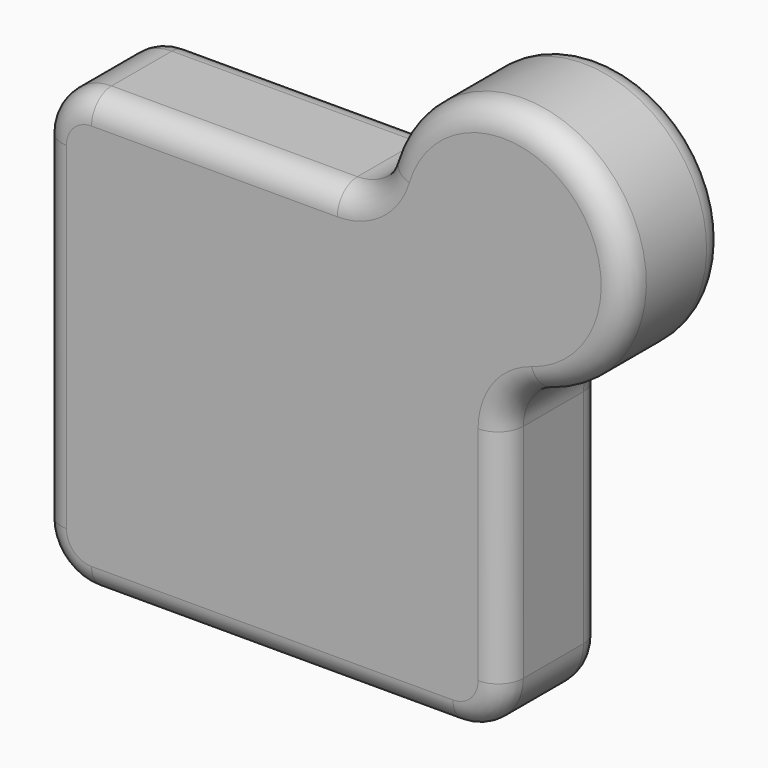
from build123d import *

# Parameters (mm, degrees)
F1_DEPTH = 25
F2_R     = 5


# Not quite as in the source:
# - the program builds the solid bodies; features that only make, move or delete a surface that nothing else refers to are left out


with BuildPart() as f1:
    # F0 (on Front) → F1 (new body)
    with BuildSketch(Plane.XZ):
        with BuildLine():
            ThreePointArc((22.5237740783, 50.7157030305), (18.9120996382, 45.5821277938), (12.9524584639, 43.6122384452))
            Line((12.9524584639, 43.6122384452), (-35.9964722395, 43.6122384452))
            ThreePointArc((-35.9964722395, 43.6122384452), (-43.0675400514, 40.6833062571), (-45.9964722395, 33.6122384452))
            Line((-45.9964722395, 33.6122384452), (-45.9964722395, -33.6122384452))
            ThreePointArc((-45.9964722395, -33.6122384452), (-43.0675400514, -40.6833062571), (-35.9964722395, -43.6122384452))
            Line((-35.9964722395, -43.6122384452), (35.9964722395, -43.6122384452))
            ThreePointArc((35.9964722395, -43.6122384452), (43.0675400514, -40.6833062571), (45.9964722395, -33.6122384452))
            Line((45.9964722395, -33.6122384452), (45.9964722395, 10.5682246696))
            ThreePointArc((45.9964722395, 10.5682246696), (47.9663615881, 16.5278658439), (53.0999368248, 20.139540284))
            ThreePointArc((53.0999368248, 20.139540284), (63.3375617105, 60.9533279162), (22.5237740783, 50.7157030305))
        make_face()
    extrude(amount=F1_DEPTH)

    # F2
    f2_edges = [f1.edges().sort_by_distance(p)[0] for p in [
        (63.337562, -25, 60.953328),
        (63.337562, 0, 60.953328),
    ]]
    fillet(f2_edges, radius=F2_R)


solid = f1.part
